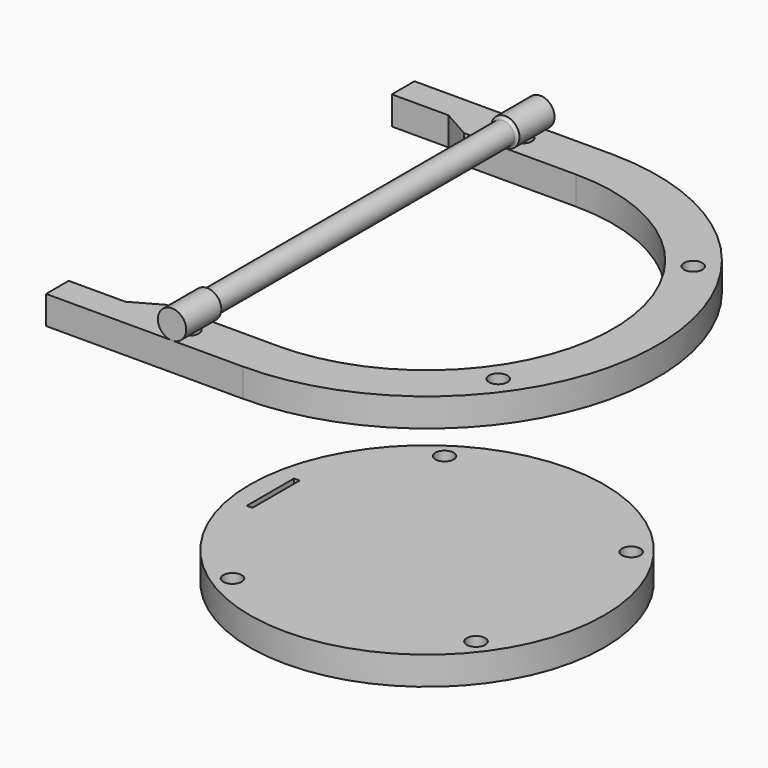
from build123d import *

# Parameters (mm, degrees)
F0_R     = 125
F0_R_2   = 6.5
F1_DEPTH = 20
F3_R     = 6.5
F4_DEPTH = 20


with BuildPart() as f1:
    # F0 (on Top) → F1 (new body)
    with BuildSketch(Plane.XY):
        Circle(F0_R)
        with Locations((-62.5, -93.5414346693)):
            Circle(F0_R_2, mode=Mode.SUBTRACT)
        Polygon((-110.5541596785, 20.8333333333), (-106.5541596785, 20.8333333333), (-106.5541596785, 0), (-106.5541596785, -20.8333333333), (-110.5541596785, -20.8333333333), (-110.5541596785, 0), align=None, mode=Mode.SUBTRACT)
        with Locations((89.2857142857, -68.4420282026)):
            Circle(F0_R_2, mode=Mode.SUBTRACT)
        with Locations((-62.5, 93.5414346693)):
            Circle(F0_R_2, mode=Mode.SUBTRACT)
        with Locations((89.2857142857, 68.4420282026)):
            Circle(F0_R_2, mode=Mode.SUBTRACT)
    extrude(amount=F1_DEPTH)


with BuildPart() as f4:
    # F3 (on offset) → F4 (new body)
    with BuildSketch(Plane.XY.offset(200)):
        with BuildLine():
            ThreePointArc((0, 131.25), (131.25, 0), (0, -131.25))
            Line((0, -131.25), (-78.8888888889, -131.25))
            Line((-78.8888888889, -131.25), (-98.8888888889, -142.5))
            Line((-98.8888888889, -142.5), (-138.8888888889, -142.5))
            Line((-138.8888888889, -142.5), (-138.8888888889, -162.5))
            Line((-138.8888888889, -162.5), (0, -162.5))
            ThreePointArc((0, -162.5), (162.5, 0), (0, 162.5))
            Line((0, 162.5), (-138.8888888889, 162.5))
            Line((-138.8888888889, 162.5), (-138.8888888889, 142.5))
            Line((-138.8888888889, 142.5), (-98.8888888889, 142.5))
            Line((-98.8888888889, 142.5), (-78.8888888889, 131.25))
            Line((-78.8888888889, 131.25), (0, 131.25))
        make_face()
        with Locations((-50, -146.875)):
            Circle(F3_R, mode=Mode.SUBTRACT)
        with Locations((119.0476190476, -86.0228459428)):
            Circle(F3_R, mode=Mode.SUBTRACT)
        with Locations((-50, 146.875)):
            Circle(F3_R, mode=Mode.SUBTRACT)
        with Locations((119.0476190476, 86.0228459428)):
            Circle(F3_R, mode=Mode.SUBTRACT)
    extrude(amount=-F4_DEPTH)


with BuildPart() as f7:
    # F6 (on offset) → F7 (revolve)
    with BuildSketch(Plane.XY.offset(210)):
        with BuildLine():
            Line((-59.9437263161, -162.5718830858), (-49.9437263161, -162.5718830858))
            Line((-49.9437263161, -162.5718830858), (-49.9437263161, 162.4281169142))
            Line((-49.9437263161, 162.4281169142), (-59.9437263161, 162.4281169142))
            Line((-59.9437263161, 162.4281169142), (-59.9437263161, 131.4281169142))
            ThreePointArc((-59.9437263161, 131.4281169142), (-58.5295127537, 130.8423304766), (-57.9437263161, 129.4281169142))
            Line((-57.9437263161, 129.4281169142), (-57.9437263161, -129.5718830858))
            ThreePointArc((-57.9437263161, -129.5718830858), (-58.5295127537, -130.9860966482), (-59.9437263161, -131.5718830858))
            Line((-59.9437263161, -131.5718830858), (-59.9437263161, -162.5718830858))
        make_face()
    revolve(axis=Axis((-49.9437263161, -0.0718830858, 210), (0, -1, 0)))


solid = Compound([f1.part, f4.part, f7.part])
